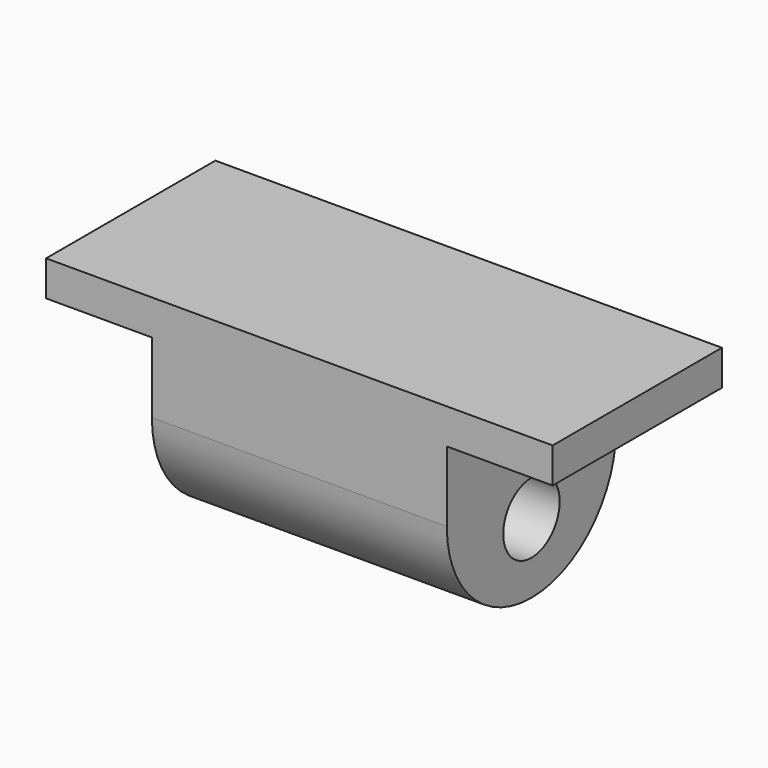
from build123d import *

# Parameters (mm, degrees)
F0_W     = 182.3974
F0_H     = 76.2
F1_DEPTH = 76.2
F2_W     = 38.1
F2_H     = 76.2
F3_DEPTH = 63.5
F4_R     = 38.09999
F5_R     = 12.7
F6_DEPTH = 144.2984


# Not quite as in the source:
# - a fillet or chamfer is up to 0.001 mm smaller than in the source, because OpenCascade refuses the exact size


with BuildPart() as f1:
    # F0 (on Top) → F1 (new body)
    with BuildSketch(Plane.XY):
        with Locations((91.1987, 38.1)):
            Rectangle(F0_W, F0_H)
    extrude(amount=F1_DEPTH)

    # F2 (on face) → F3 (cut)
    with BuildSketch(Plane(origin=(0, 0, 0), x_dir=(1, 0, 0), z_dir=(0, 0, -1))):
        with Locations((163.3474, -38.1)):
            Rectangle(F2_W, F2_H)
        with Locations((19.05, -38.1)):
            Rectangle(F2_W, F2_H)
    extrude(amount=-F3_DEPTH, mode=Mode.SUBTRACT)

    # F4 (radius 38.1 in the source; OpenCascade refuses exactly that, so slightly less here)
    f4_edges = [f1.edges().sort_by_distance(p)[0] for p in [
        (91.1987, 0, 0),
        (91.1987, 76.2, 0),
    ]]
    fillet(f4_edges, radius=F4_R)

    # F5 (on face) → F6 (cut, through all)
    with BuildSketch(Plane.YZ.offset(144.2974)):
        with Locations((38.1, 25.4)):
            Circle(F5_R)
    extrude(amount=-F6_DEPTH, mode=Mode.SUBTRACT)


solid = f1.part
